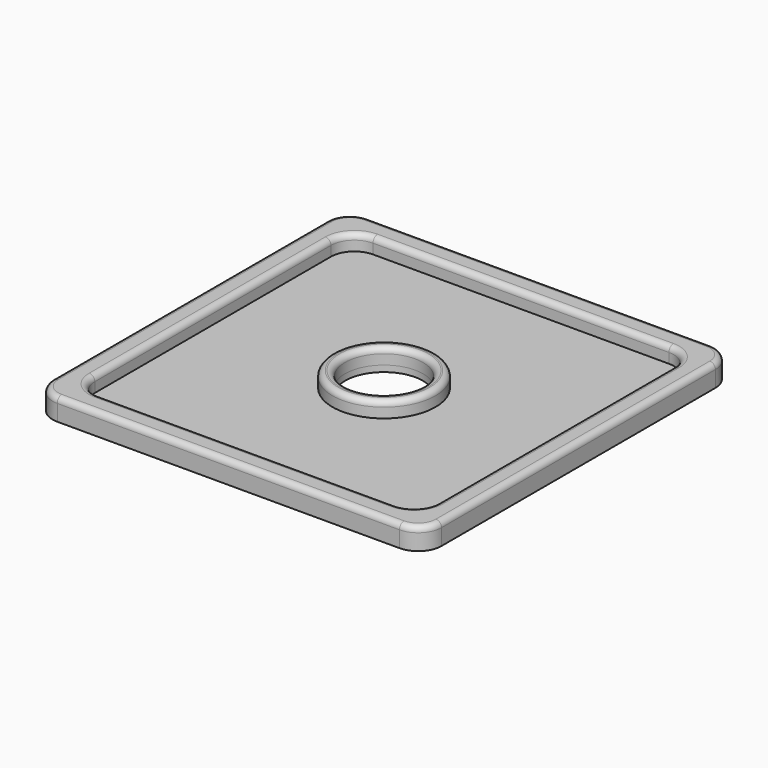
from build123d import *

# Parameters (mm, degrees)
F1_DEPTH = 0.508
F2_DEPTH = 0.2032
F3_R     = 0.762
F5_R     = 1.6807405663
F6_DEPTH = 0.508
F7_D     = 2.54
F7_DEPTH = 0.509
F8_D     = 2.54
F8_DEPTH = 0.2042
F9_R     = 0.1839630735


with BuildPart() as f1:
    # F0 (on Top) → F1 (new body)
    with BuildSketch(Plane.XY):
        Polygon((-12.694504112, 12.6988124102), (-12.694504112, 6.3494062051), (-11.9335213676, 6.3494062051), (-11.9335213676, 11.9331842288), (-6.347252056, 11.9331842288), (-6.347252056, 12.6988124102), align=None)
        Polygon((-0.7515071775, 6.3494062051), (0, 6.3494062051), (0, 12.6988124102), (-6.347252056, 12.6988124102), (-6.347252056, 11.9331842288), (-0.7515071775, 11.9331842288), align=None)
        Polygon((-6.347252056, 0), (0, 0), (0, 6.3494062051), (-0.7515071775, 6.3494062051), (-0.7515071775, 0.7721490692), (-6.347252056, 0.7721490692), align=None)
        Polygon((-12.694504112, 0), (-6.347252056, 0), (-6.347252056, 0.7721490692), (-11.9335213676, 0.7721490692), (-11.9335213676, 6.3494062051), (-12.694504112, 6.3494062051), align=None)
    extrude(amount=F1_DEPTH)

    # F0 (on Top) → F2 (join)
    with BuildSketch(Plane.XY):
        Polygon((-11.9335213676, 0.7721490692), (-6.347252056, 0.7721490692), (-0.7515071775, 0.7721490692), (-0.7515071775, 6.3494062051), (-0.7515071775, 11.9331842288), (-6.347252056, 11.9331842288), (-11.9335213676, 11.9331842288), (-11.9335213676, 6.3494062051), align=None)
        Polygon((-12.694504112, 12.6988124102), (-12.694504112, 6.3494062051), (-11.9335213676, 6.3494062051), (-11.9335213676, 11.9331842288), (-6.347252056, 11.9331842288), (-6.347252056, 12.6988124102), align=None)
        Polygon((-12.694504112, 0), (-6.347252056, 0), (-6.347252056, 0.7721490692), (-11.9335213676, 0.7721490692), (-11.9335213676, 6.3494062051), (-12.694504112, 6.3494062051), align=None)
        Polygon((-6.347252056, 0), (0, 0), (0, 6.3494062051), (-0.7515071775, 6.3494062051), (-0.7515071775, 0.7721490692), (-6.347252056, 0.7721490692), align=None)
        Polygon((-0.7515071775, 6.3494062051), (0, 6.3494062051), (0, 12.6988124102), (-6.347252056, 12.6988124102), (-6.347252056, 11.9331842288), (-0.7515071775, 11.9331842288), align=None)
    extrude(amount=-F2_DEPTH)

    # F3
    f3_edges = [f1.edges().sort_by_distance(p)[0] for p in [
        (0, 0, 0.1524),
        (0, 12.698812, 0.1524),
        (-12.694504, 12.698812, 0.1524),
        (-12.694504, 0, 0.1524),
        (-11.933521, 11.933184, 0.254),
        (-11.933521, 0.772149, 0.254),
        (-0.751507, 11.933184, 0.254),
        (-0.751507, 0.772149, 0.254),
    ]]
    fillet(f3_edges, radius=F3_R)

    # F5 (on offset) → F6 (join)
    with BuildSketch(Plane.XY):
        with Locations((-6.3472064212, 6.3493414782)):
            Circle(F5_R)
    extrude(amount=F6_DEPTH)

    # F7 (through all, one way)
    with BuildSketch(Plane(origin=(0, 0, 0), x_dir=(1, 0, 0), z_dir=(0, 0, -1))):
        with Locations((-6.3472064212, -6.3493414782)):
            Circle(F7_D / 2)
    extrude(amount=-F7_DEPTH, mode=Mode.SUBTRACT)

    # F8 (through all, one way)
    with BuildSketch(Plane.XY):
        with Locations((-6.347252056, 6.3494062051)):
            Circle(F8_D / 2)
    extrude(amount=-F8_DEPTH, mode=Mode.SUBTRACT)

    # F9
    f9_edges = [f1.edges().sort_by_distance(p)[0] for p in [
        (-8.027947, 6.349341, 0.508),
        (0, 6.349406, 0.508),
        (-0.751507, 6.352667, 0.508),
        (-12.694504, 6.349406, 0.508),
        (-12.471319, 12.475628, 0.508),
        (-12.471319, 0.223185, 0.508),
        (-6.347252, 12.698812, 0.508),
        (-6.347252, 0, 0.508),
        (-0.223185, 12.475628, 0.508),
        (-0.223185, 0.223185, 0.508),
        (-6.342514, 11.933184, 0.508),
        (-11.710337, 11.71, 0.508),
        (-0.974692, 11.71, 0.508),
        (-11.933521, 6.352667, 0.508),
        (-11.710337, 0.995334, 0.508),
        (-0.974692, 0.995334, 0.508),
        (-6.342514, 0.772149, 0.508),
        (-7.617206, 6.349341, 0.508),
    ]]
    fillet(f9_edges, radius=F9_R)


solid = f1.part
